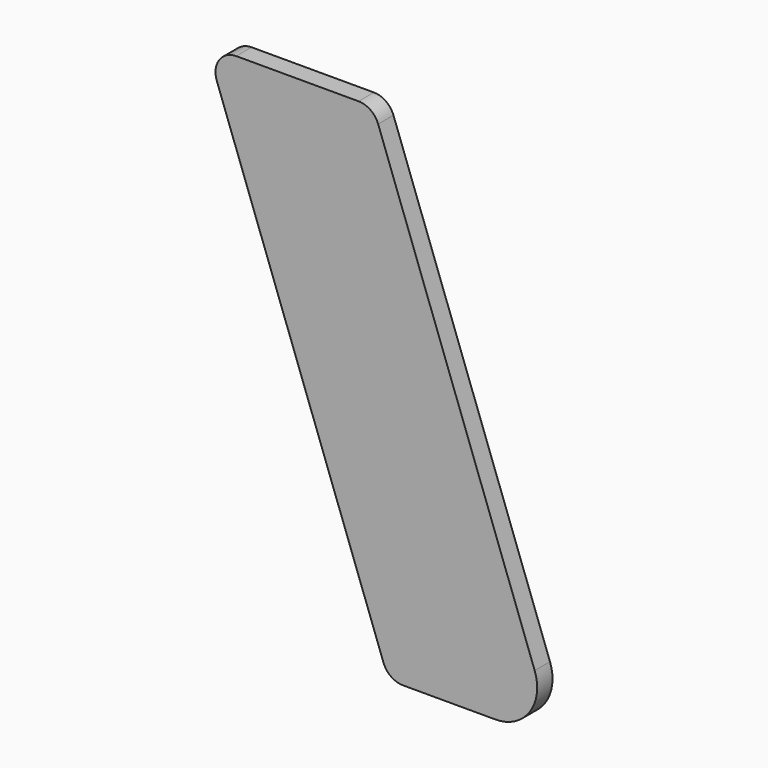
from build123d import *

# Parameters (mm, degrees)
F1_DEPTH = 5.842
F2_R     = 6.35
F3_R     = 12.7


# Not quite as in the source:
# - a length typed as a fraction of an inch, garbled in the dataset ("3 / 203.2 mm" for 3/8 in), is restored


with BuildPart() as f1:
    # F0 (on Front) → F1 (new body)
    with BuildSketch(Plane.XZ):
        Polygon((50.8, 0), (0, 0), (55.4690637022, -152.4), (106.2690637022, -152.4), align=None)
    extrude(amount=F1_DEPTH)

    # F2
    f2_edges = [f1.edges().sort_by_distance(p)[0] for p in [
        (55.469064, -2.921, -152.4),
        (50.8, -2.921, 0),
        (0, -2.921, 0),
    ]]
    fillet(f2_edges, radius=F2_R)

    # F3
    f3_edges = [f1.edges().sort_by_distance(p)[0] for p in [
        (106.269064, -2.921, -152.4),
    ]]
    fillet(f3_edges, radius=F3_R)


solid = f1.part
